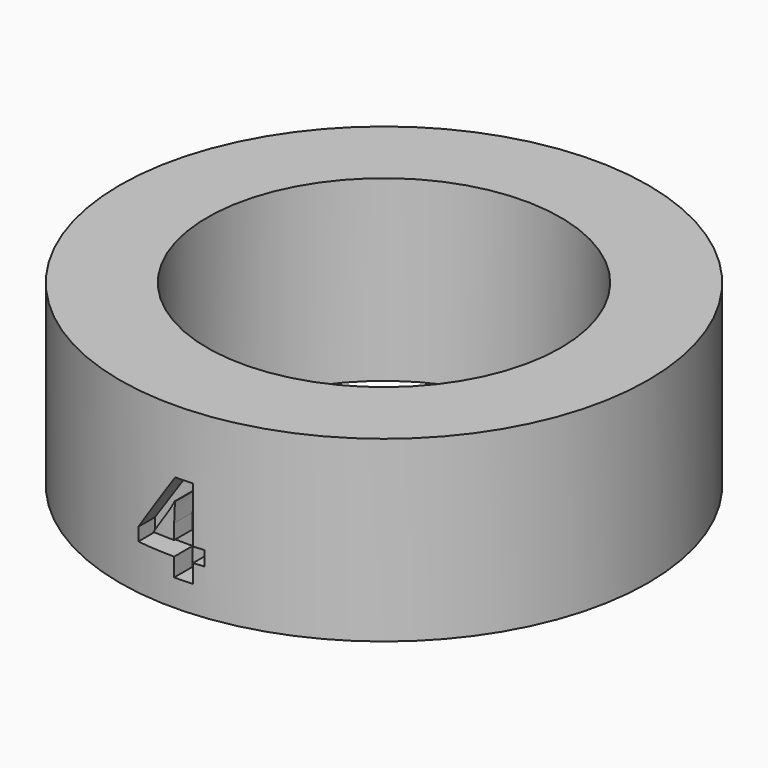
from build123d import *

# Parameters (mm, degrees)
F0_R         = 14.8
F0_R_2       = 9.9
F1_DEPTH     = 10
F3_TEXT_SIZE = 6.9444444444
F4_DEPTH     = 1.5


# Not quite as in the source:
# - Text() gives the source's letters only with a copy of the font that has no kerning and outlines rounded to 1/6400 em; it was checked with that copy


with BuildPart() as f1:
    # F0 (on Top) → F1 (new body)
    with BuildSketch(Plane.XY):
        Circle(F0_R)
        Circle(F0_R_2, mode=Mode.SUBTRACT)
    extrude(amount=F1_DEPTH)

    # F3 (on offset) → F4 (cut)
    with BuildSketch(Plane.XZ.offset(15)):
        with Locations((-2.1527777778, 1.500000013)):
            Text('4', F3_TEXT_SIZE, font='Open Sans', font_style=FontStyle.BOLD, text_align=(TextAlign.LEFT, TextAlign.BOTTOM))
    extrude(amount=-F4_DEPTH, mode=Mode.SUBTRACT)


solid = f1.part
